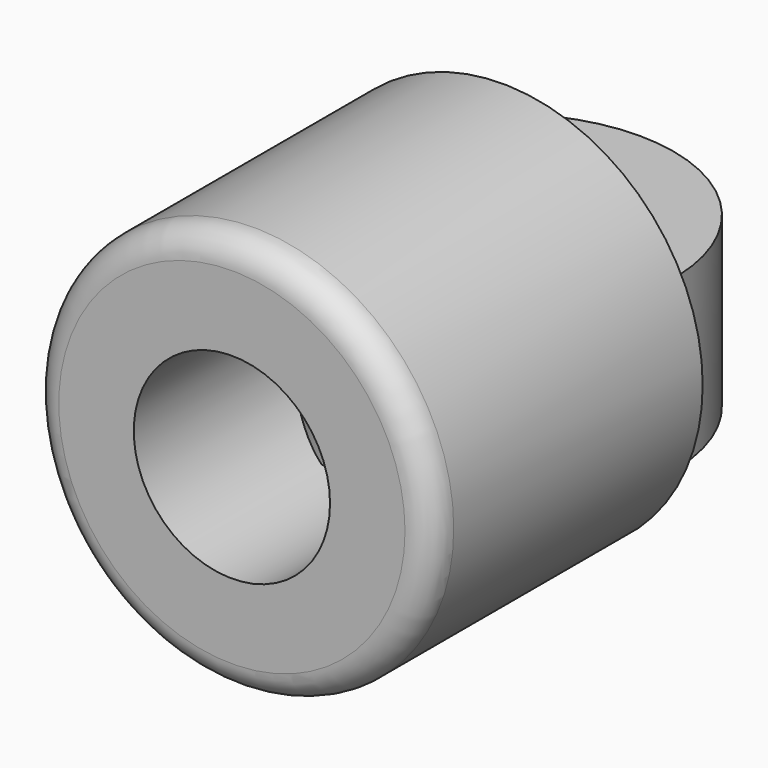
from build123d import *

# Parameters (mm, degrees)
F0_R         = 150.3237387913
F0_R_2       = 73.6926609148
F1_DEPTH     = 254
F2_R         = 20.32
F3_R         = 112.9256404591
F3_R_2       = 87.0757104376
F4_DEPTH     = 25.4
F5_R         = 128.6901964601
F6_DEPTH     = 63.5
F7_T4_DEPTH  = 60.7095224794
F7_S5_R      = 128.6901964601
F7_T6_DEPTH  = 32
F7_T10_DEPTH = 60.7095224794
F7_S11_R     = 128.6901964601
F7_T12_DEPTH = 32
F7_T16_DEPTH = 60.7095224794
F7_S17_R     = 128.6901964601
F7_T18_DEPTH = 32
F7_T22_DEPTH = 60.7095224794
F7_S23_R     = 128.6901964601
F7_T24_DEPTH = 32


# Not quite as in the source:
# - a fillet or chamfer that OpenCascade refuses, or shapes differently, is made with other operations: its cross-section is extruded or revolved along the edge and cut away or added


with BuildPart() as f1:
    # F0 (on Front) → F1 (new body)
    with BuildSketch(Plane.XZ):
        Circle(F0_R)
        Circle(F0_R_2, mode=Mode.SUBTRACT)
    extrude(amount=F1_DEPTH)

    # F2
    f2_edges = [f1.edges().sort_by_distance(p)[0] for p in [
        (-150.323739, -254, 0),
    ]]
    fillet(f2_edges, radius=F2_R)

    # F3 (on face) → F4 (join)
    with BuildSketch(Plane(origin=(0, 0, 0), x_dir=(-1, 0, 0), z_dir=(0, 1, 0))):
        Circle(F3_R)
        Circle(F3_R_2, mode=Mode.SUBTRACT)
    extrude(amount=F4_DEPTH)

    # F5 (on Top) → F6 (join, symmetric)
    with BuildSketch(Plane.XY):
        Circle(F5_R)
    extrude(amount=F6_DEPTH, both=True)

    # F7: fillet of radius 5.08 on 4 edges, made by hand


with BuildPart() as f7_tool2:
    # F7_s3 → F7_t4 (new body)
    with BuildSketch(Plane.YZ.offset(-80.6806739807)):
        with BuildLine():
            ThreePointArc((0, -68.58), (1.4878975516, -64.9878975516), (5.08, -63.5))
            Line((5.08, -63.5), (0, -63.5))
            Line((0, -63.5), (0, -68.58))
        make_face()
    extrude(amount=-F7_T4_DEPTH)

    # F7_s5 → F7_t6 (intersect, symmetric)
    with BuildSketch(Plane.XY.offset(-66)):
        Circle(F7_S5_R)
    extrude(amount=F7_T6_DEPTH, both=True, mode=Mode.INTERSECT)


with BuildPart() as f1_1:
    add(f1.part)

    # F7_t1: union F7_tool2
    add(f7_tool2.part)


with BuildPart() as f7_tool8:
    # F7_s9 → F7_t10 (new body)
    with BuildSketch(Plane.YZ.offset(141.3901964601)):
        with BuildLine():
            ThreePointArc((0, -68.58), (1.4878975516, -64.9878975516), (5.08, -63.5))
            Line((5.08, -63.5), (0, -63.5))
            Line((0, -63.5), (0, -68.58))
        make_face()
    extrude(amount=-F7_T10_DEPTH)

    # F7_s11 → F7_t12 (intersect, symmetric)
    with BuildSketch(Plane.XY.offset(-66)):
        Circle(F7_S11_R)
    extrude(amount=F7_T12_DEPTH, both=True, mode=Mode.INTERSECT)


with BuildPart() as f1_2:
    add(f1_1.part)

    # F7_t7: union F7_tool8
    add(f7_tool8.part)


with BuildPart() as f7_tool14:
    # F7_s15 → F7_t16 (new body)
    with BuildSketch(Plane.YZ.offset(-80.6806739807)):
        with BuildLine():
            ThreePointArc((0, 68.58), (1.4878975516, 64.9878975516), (5.08, 63.5))
            Line((5.08, 63.5), (0, 63.5))
            Line((0, 63.5), (0, 68.58))
        make_face()
    extrude(amount=-F7_T16_DEPTH)

    # F7_s17 → F7_t18 (intersect, symmetric)
    with BuildSketch(Plane.XY.offset(66)):
        Circle(F7_S17_R)
    extrude(amount=F7_T18_DEPTH, both=True, mode=Mode.INTERSECT)


with BuildPart() as f1_3:
    add(f1_2.part)

    # F7_t13: union F7_tool14
    add(f7_tool14.part)


with BuildPart() as f7_tool20:
    # F7_s21 → F7_t22 (new body)
    with BuildSketch(Plane.YZ.offset(141.3901964601)):
        with BuildLine():
            ThreePointArc((0, 68.58), (1.4878975516, 64.9878975516), (5.08, 63.5))
            Line((5.08, 63.5), (0, 63.5))
            Line((0, 63.5), (0, 68.58))
        make_face()
    extrude(amount=-F7_T22_DEPTH)

    # F7_s23 → F7_t24 (intersect, symmetric)
    with BuildSketch(Plane.XY.offset(66)):
        Circle(F7_S23_R)
    extrude(amount=F7_T24_DEPTH, both=True, mode=Mode.INTERSECT)


with BuildPart() as f1_4:
    add(f1_3.part)

    # F7_t19: union F7_tool20
    add(f7_tool20.part)


solid = f1_4.part
